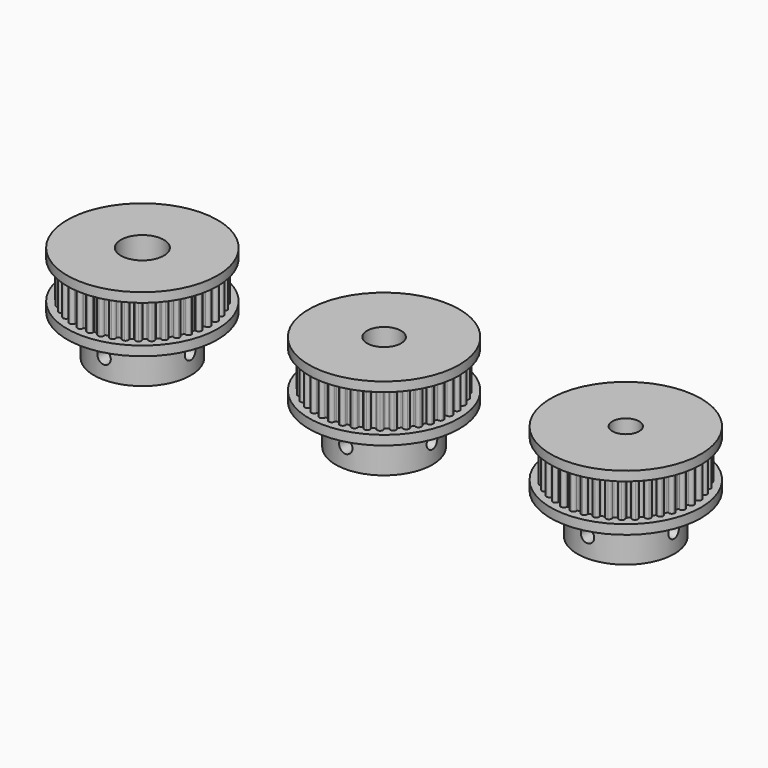
from build123d import *

# Parameters (mm, degrees)
F3_DEPTH        = 7
F3_COPIES_COUNT = 40
F7_D            = 2.5
F7_DEPTH        = 10
F7_START        = 0.0872284
F7_TIP          = 0.7510757738
F7_COPIES_COUNT = 2
F7_COPIES_ANGLE = 270
F11_D           = 8
F12_D           = 6.35
F13_D           = 5


# Not quite as in the source:
# - a pattern or mirror of a feature is missing from the dataset's text; its kind, count and spacing are read off the source's solid


with BuildPart() as f1:
    # F0 (on Front) → F1 (revolve)
    with BuildSketch(Plane.XZ):
        Polygon((0, 16.25), (0, 0), (9, 0), (9, 7.5), (14, 7.5), (14, 9.25), (12.7323954474, 9.25), (12.7323954474, 16.25), align=None)
    revolve(axis=Axis((0, 0, 9), (0, 0, -1)))

    # F2 (on face) → F3 (cut, through all)
    with BuildSketch(Plane.XY.offset(16.25)):
        with BuildLine():
            ThreePointArc((0.5533902288, 12.1166132454), (0.5926491162, 12.0107394812), (0.6946234896, 11.9622447251))
            ThreePointArc((0.6946234896, 11.9622447251), (0.9401279115, 11.9454577211), (1.1852358324, 11.9236326964))
            ThreePointArc((1.1852358324, 11.9236326964), (1.2935409833, 11.9555780949), (1.3488788344, 12.0540069344))
            Line((1.3488788344, 12.0540069344), (1.3543829299, 12.0973650514))
            ThreePointArc((1.3543829299, 12.0973650514), (1.5718655872, 12.4713974186), (1.9917854705, 12.5756385312))
            ThreePointArc((1.9917854705, 12.5756385312), (0.9989722332, 12.6931457214), (0, 12.7323954474))
            ThreePointArc((0, 12.7323954474), (0.39844307, 12.5637477735), (0.5547366016, 12.1602985823))
            Line((0.5547366016, 12.1602985823), (0.5533902288, 12.1166132454))
        make_face()
    f3 = extrude(amount=-F3_DEPTH, mode=Mode.SUBTRACT)

    # F3_copies: F3 ×40 about axis
    f3_copies_axis = Axis((0, 0, 0), (0, 0, 1))
    for i in range(1, F3_COPIES_COUNT):
        add(f3.rotate(f3_copies_axis, i * 360 / F3_COPIES_COUNT), mode=Mode.SUBTRACT)

    # F0 (on Front) → F4 (revolve)
    with BuildSketch(Plane.XZ):
        Polygon((0, 18), (0, 16.25), (12.7323954474, 16.25), (14, 16.25), (14, 18), align=None)
    revolve(axis=Axis((0, 0, 9), (0, 0, -1)))

    # F7
    # its depths count from where the whole tool has entered the part; down to there all is cleared
    with Locations(Plane.YZ.offset(9).offset(-F7_START)):
        with Locations((0, 3.75)):
            f7 = Hole(F7_D / 2, depth=F7_DEPTH)
            with Locations((0, 0, -(F7_DEPTH + F7_TIP / 2))):  # 118° drill point
                Cone(0, F7_D / 2, F7_TIP, mode=Mode.SUBTRACT)

    # F7_copies: F7 ×2 about axis
    f7_copies_axis = Axis((0, 0, 0), (0, 0, 1))
    for i in range(1, F7_COPIES_COUNT):
        add(f7.rotate(f7_copies_axis, i * F7_COPIES_ANGLE / (F7_COPIES_COUNT - 1)), mode=Mode.SUBTRACT)


with BuildPart() as f8_1:
    # F8: copy of F1
    add(f1.part.moved(Location((45, 0, 0))))


with BuildPart() as f9_1:
    # F9: copy of F8_1
    add(f8_1.part.moved(Location((45, 0, 0))))

    # F13 (through all)
    with Locations(Plane.XY.offset(18)):
        with Locations((90, 0)):
            Hole(F13_D / 2)


with BuildPart() as f1_1:
    add(f1.part)

    # F11 (through all)
    with Locations(Plane.XY.offset(18)):
        with Locations((0, 0)):
            Hole(F11_D / 2)


with BuildPart() as f8_1_1:
    add(f8_1.part)

    # F12 (through all)
    with Locations(Plane.XY.offset(18)):
        with Locations((45, 0)):
            Hole(F12_D / 2)


solid = Compound([f9_1.part, f1_1.part, f8_1_1.part])
